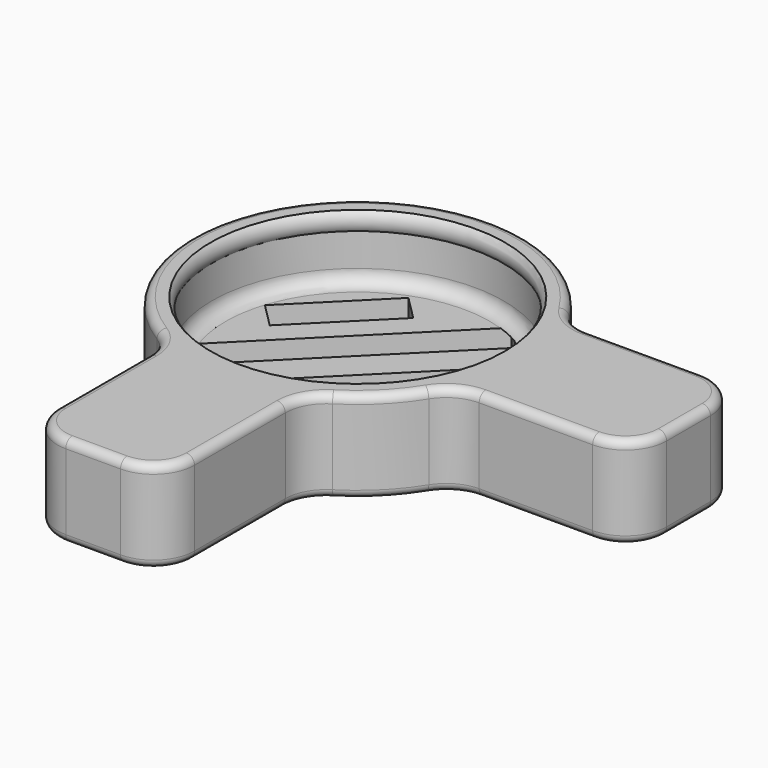
from build123d import *

# Parameters (mm, degrees)
F3_DEPTH = 8.5269614104
F4_R     = 3.81
F5_R     = 0.762
F7_DEPTH = 25.4


with BuildPart() as f1:
    # F0 (on Front) → F1 (revolve)
    with BuildSketch(Plane.XZ):
        with BuildLine():
            Line((15.4305, 0), (15.4305, 6.7130385896))
            ThreePointArc((15.4305, 6.7130385896), (14.4451376493, 6.3536610654), (13.5255, 6.858))
            Line((13.5255, 6.858), (13.5255, 3.81))
            ThreePointArc((13.5255, 3.81), (13.1535256121, 2.9119743879), (12.2555, 2.54))
            Line((12.2555, 2.54), (0, 2.54))
            Line((0, 2.54), (0, 0))
            Line((0, 0), (15.4305, 0))
        make_face()
        with BuildLine():
            ThreePointArc((13.5255, 6.858), (14.4451376493, 6.3536610654), (15.4305, 6.7130385896))
            Line((15.4305, 6.7130385896), (15.4305, 8.5269614104))
            Line((15.4305, 8.5269614104), (13.6525, 8.5269614104))
            ThreePointArc((13.6525, 8.5269614104), (13.2751610654, 7.7163623507), (13.5255, 6.858))
        make_face()
    revolve(axis=Axis((0, 0, 4.2298094004), (0, 0, -1)))

    # F2 (on face) → F3 (join, through all)
    with BuildSketch(Plane.XY.offset(8.5269614104)):
        with BuildLine():
            Line((30.6705, -6.35), (30.6705, 6.35))
            Line((30.6705, 6.35), (14.0633506054, 6.35))
            ThreePointArc((14.0633506054, 6.35), (15.4305, 0), (14.0633506054, -6.35))
            Line((14.0633506054, -6.35), (30.6705, -6.35))
        make_face()
        with BuildLine():
            Line((-6.35, -30.6705), (6.35, -30.6705))
            Line((6.35, -30.6705), (6.35, -14.0633506054))
            ThreePointArc((6.35, -14.0633506054), (0, -15.4305), (-6.35, -14.0633506054))
            Line((-6.35, -14.0633506054), (-6.35, -30.6705))
        make_face()
    extrude(amount=-F3_DEPTH)

    # F4
    f4_edges = [f1.edges().sort_by_distance(p)[0] for p in [
        (-6.35, -30.6705, 4.263481),
        (-6.35, -14.063351, 4.263481),
        (6.35, -30.6705, 4.263481),
        (6.35, -14.063351, 4.263481),
        (14.063351, -6.35, 4.263481),
        (30.6705, -6.35, 4.263481),
        (30.6705, 6.35, 4.263481),
        (14.063351, 6.35, 4.263481),
    ]]
    fillet(f4_edges, radius=F4_R)

    # F5
    f5_edges = [f1.edges().sort_by_distance(p)[0] for p in [
        (0, -30.6705, 8.526961),
        (0, -30.6705, 0),
    ]]
    fillet(f5_edges, radius=F5_R)

    # F6 (on face) → F7 (cut)
    with BuildSketch(Plane.XY.offset(2.54)):
        Polygon((2.7523231475, -11.7213891216), (11.76669461, -2.7070176591), (9.5216305797, -0.4619536288), (0.5072591172, -9.4763250914), align=None)
        Polygon((-4.5321477931, -10.0819004043), (9.9724980907, 4.4227454795), (7.7274340604, 6.6678095097), (-6.7772118234, -7.836836374), align=None)
        Polygon((-9.6811759284, -6.5377472694), (6.7586679854, 9.9020966443), (4.5136039551, 12.1471606746), (-11.9262399586, -4.2926832391), align=None)
        Polygon((-9.3679427371, 1.5062135006), (-1.974369983, 8.8997862547), (-4.2194340133, 11.144850285), (-11.6130067674, 3.7512775309), align=None)
    extrude(amount=-F7_DEPTH, mode=Mode.SUBTRACT)


solid = f1.part
